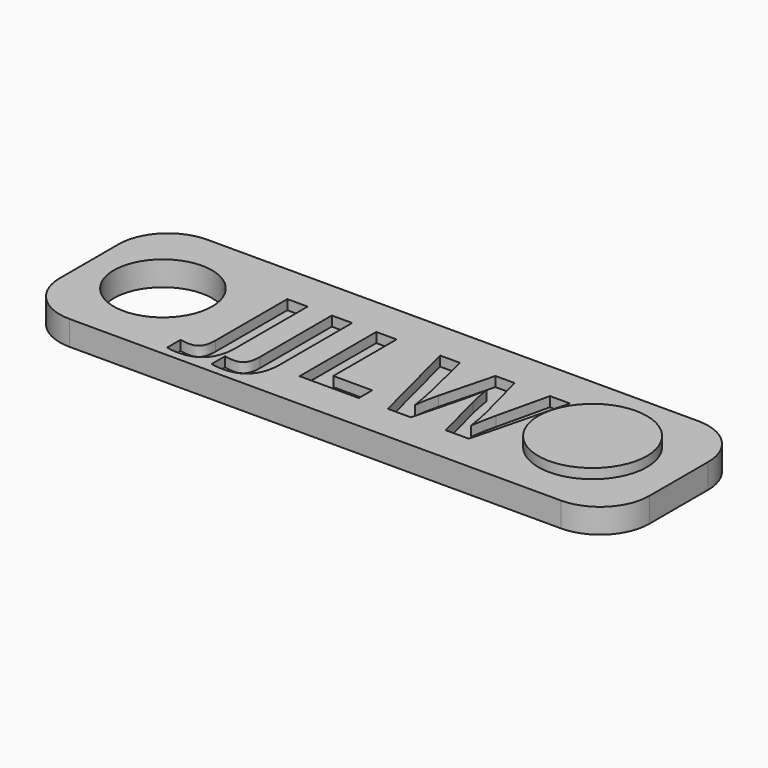
from build123d import *

# Parameters (mm, degrees)
F0_W         = 120
F0_H         = 35
F1_DEPTH     = 5
F2_R         = 10
F3_R         = 10
F4_DEPTH     = 5
F5_TEXT_SIZE = 27.34375238
F6_DEPTH     = 2
F7_R         = 11.0542028091
F8_DEPTH     = 2


# Not quite as in the source:
# - Text() gives the source's letters only with a copy of the font that has no kerning and outlines rounded to 1/6400 em; it was checked with that copy


with BuildPart() as f1:
    # F0 (on Top) → F1 (new body)
    with BuildSketch(Plane.XY):
        Rectangle(F0_W, F0_H)
    extrude(amount=F1_DEPTH)

    # F2
    f2_edges = [f1.edges().sort_by_distance(p)[0] for p in [
        (-60, -17.5, 2.5),
        (-60, 17.5, 2.5),
        (60, 17.5, 2.5),
        (60, -17.5, 2.5),
    ]]
    fillet(f2_edges, radius=F2_R)

    # F3 (on face) → F4 (cut)
    with BuildSketch(Plane.XY.offset(5)):
        with Locations((-45, 0)):
            Circle(F3_R)
    extrude(amount=-F4_DEPTH, mode=Mode.SUBTRACT)

    # F5 (on face) → F6 (cut)
    with BuildSketch(Plane.XY.offset(5)):
        with Locations((-29.7242663801, -10.0367655978)):
            Text('JJLW', F5_TEXT_SIZE, font='Open Sans', font_style=FontStyle.BOLD, text_align=(TextAlign.LEFT, TextAlign.BOTTOM))
    extrude(amount=-F6_DEPTH, mode=Mode.SUBTRACT)

    # F7 (on face) → F8 (join)
    with BuildSketch(Plane.XY.offset(5)):
        with Locations((42.4632355571, 0)):
            Circle(F7_R)
    extrude(amount=F8_DEPTH)


solid = f1.part
